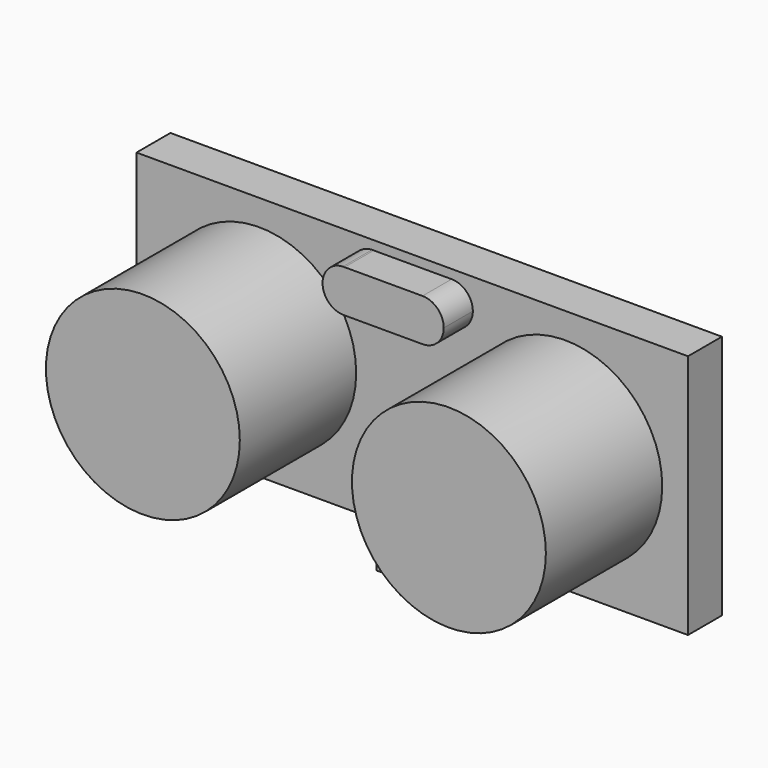
from build123d import *

# Parameters (mm, degrees)
F0_R     = 8
F0_W     = 10.5
F0_H     = 3
F1_DEPTH = 3.5
F2_DEPTH = 15.5
F3_DEPTH = 6.5
F0_H_2   = 6
F4_DEPTH = 2


with BuildPart() as f1:
    # F0 (on Front) → F1 (new body)
    with BuildSketch(Plane.XZ):
        Polygon((22.75, 10.125), (-22.75, 10.125), (-22.75, -10.125), (-5.75, -10.125), (-5.75, -7.125), (4.75, -7.125), (4.75, -10.125), (22.75, -10.125), align=None)
        with Locations((-12.625, 0)):
            Circle(F0_R, mode=Mode.SUBTRACT)
        with Locations((12.625, 0)):
            Circle(F0_R, mode=Mode.SUBTRACT)
        with BuildLine():
            ThreePointArc((-3.25, 5.8816159739), (-4.9996694778, 7.5976054108), (-3.3180082792, 9.38029401))
            ThreePointArc((-3.3180082792, 9.38029401), (-3.2503522375, 9.3816159385), (-3.1826956692, 9.3803212456))
            Line((-3.1826956692, 9.3803212456), (3.2496477625, 9.3816159385))
            ThreePointArc((3.2496477625, 9.3816159385), (4.487312326, 8.8691773695), (5, 7.6316159739))
            ThreePointArc((5, 7.6316159739), (4.4874368671, 6.3941791069), (3.25, 5.8816159739))
            Line((3.25, 5.8816159739), (-3.25, 5.8816159739))
        make_face(mode=Mode.SUBTRACT)
        with Locations((-0.5, -8.625)):
            Rectangle(F0_W, F0_H)
        with Locations((-12.625, 0)):
            Circle(F0_R)
        with Locations((12.625, 0)):
            Circle(F0_R)
        with BuildLine():
            ThreePointArc((-3.1826956692, 9.3803212456), (-3.2503522375, 9.3816159385), (-3.3180082792, 9.38029401))
            Line((-3.3180082792, 9.38029401), (-3.1826956692, 9.3803212456))
        make_face()
    extrude(amount=F1_DEPTH)

    # F0 (on Front) → F2 (join)
    with BuildSketch(Plane.XZ):
        with Locations((-12.625, 0)):
            Circle(F0_R)
        with Locations((12.625, 0)):
            Circle(F0_R)
    extrude(amount=F2_DEPTH)

    # F0 (on Front) → F3 (join)
    with BuildSketch(Plane.XZ):
        with BuildLine():
            Line((3.2496477625, 9.3816159385), (-3.1826956692, 9.3803212456))
            ThreePointArc((-3.1826956692, 9.3803212456), (-1.988991955, 8.8450238652), (-1.5, 7.6316159739))
            Line((-1.5, 7.6316159739), (1.5, 7.6316159739))
            ThreePointArc((1.5, 7.6316159739), (2.0124386044, 8.8689283), (3.2496477625, 9.3816159385))
        make_face()
        with BuildLine():
            ThreePointArc((-1.5, 7.6316159739), (-2.0125631329, 6.3941791069), (-3.25, 5.8816159739))
            Line((-3.25, 5.8816159739), (3.25, 5.8816159739))
            ThreePointArc((3.25, 5.8816159739), (2.0125631329, 6.3941791069), (1.5, 7.6316159739))
            Line((1.5, 7.6316159739), (-1.5, 7.6316159739))
        make_face()
        with BuildLine():
            Line((-3.1826956692, 9.3803212456), (-3.3180082792, 9.38029401))
            ThreePointArc((-3.3180082792, 9.38029401), (-4.9996694778, 7.5976054108), (-3.25, 5.8816159739))
            ThreePointArc((-3.25, 5.8816159739), (-2.0125631329, 6.3941791069), (-1.5, 7.6316159739))
            ThreePointArc((-1.5, 7.6316159739), (-1.988991955, 8.8450238652), (-3.1826956692, 9.3803212456))
        make_face()
        with BuildLine():
            ThreePointArc((1.5, 7.6316159739), (2.0125631329, 6.3941791069), (3.25, 5.8816159739))
            ThreePointArc((3.25, 5.8816159739), (4.4874368671, 6.3941791069), (5, 7.6316159739))
            ThreePointArc((5, 7.6316159739), (4.487312326, 8.8691773695), (3.2496477625, 9.3816159385))
            ThreePointArc((3.2496477625, 9.3816159385), (2.0124386044, 8.8689283), (1.5, 7.6316159739))
        make_face()
    extrude(amount=F3_DEPTH)

    # F0 (on Front) → F4 (join)
    with BuildSketch(Plane.XZ):
        with Locations((-0.5, -8.625)):
            Rectangle(F0_W, F0_H)
        with Locations((-0.5, -13.125)):
            Rectangle(F0_W, F0_H_2)
    extrude(amount=-F4_DEPTH)


solid = f1.part
